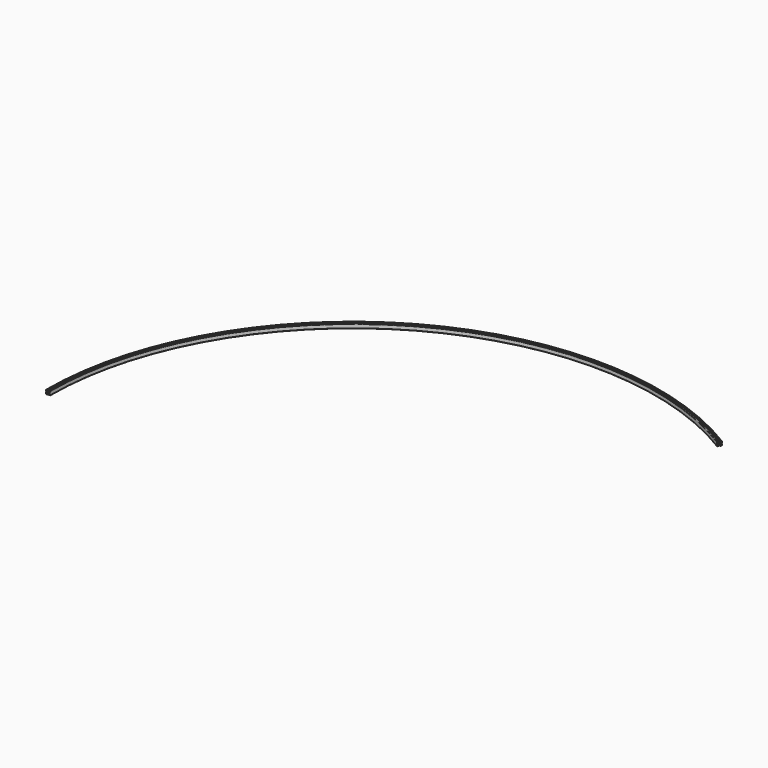
from build123d import *


# Not quite as in the source:
# - ends of sketch curves that miss each other by under 0.0002 mm in the source are joined


with BuildPart() as f2:
    # F2: sweep along a path in F1
    with BuildLine(Plane.XY) as f2_path:
        ThreePointArc((0, 0), (1542.5596027822, 2633.9267022203), (4594.4171342179, 2577.132260378))
    # F0 (on Front) → F2 (sweep)
    with BuildSketch(Plane.XZ):
        with BuildLine():
            Line((20, -17.173511), (20, 17))
            ThreePointArc((20, 17), (19.1213203436, 19.1213203436), (17, 20))
            Line((17, 20), (4.1, 20))
            Line((4.1, 20), (4.1, 17))
            Line((4.1, 17), (10.5, 17))
            Line((10.5, 17), (10.5, 12.662742))
            ThreePointArc((10.5, 12.662742), (10.378207252, 12.0504485082), (10.0313708499, 11.5313711501))
            Line((10.0313708499, 11.5313711501), (8.171573, 9.671573))
            ThreePointArc((8.171573, 9.671573), (6.8738797295, 8.80448187), (5.343146, 8.5))
            Line((5.343146, 8.5), (-5.343146, 8.5))
            ThreePointArc((-5.343146, 8.5), (-6.8738797295, 8.80448187), (-8.1715731247, 9.6715728753))
            Line((-8.1715731247, 9.6715728753), (-10.031371, 11.531371))
            ThreePointArc((-10.031371, 11.531371), (-10.378207252, 12.0504485082), (-10.5, 12.662742))
            Line((-10.5, 12.662742), (-10.5, 17))
            Line((-10.5, 17), (-4.1, 17))
            Line((-4.1, 17), (-4.1, 20))
            Line((-4.1, 20), (-17, 20))
            ThreePointArc((-17, 20), (-19.1213203436, 19.1213203436), (-20, 17))
            Line((-20, 17), (-20, 4.1))
            Line((-20, 4.1), (-17, 4.1))
            Line((-17, 4.1), (-17, 10.5))
            Line((-17, 10.5), (-12.662742, 10.5))
            ThreePointArc((-12.662742, 10.5), (-12.0504485082, 10.378207252), (-11.5313711501, 10.0313708499))
            Line((-11.5313711501, 10.0313708499), (-9.671573, 8.171573))
            ThreePointArc((-9.671573, 8.171573), (-8.80448187, 6.8738797295), (-8.5, 5.343146))
            Line((-8.5, 5.343146), (-8.5, -5.343146))
            ThreePointArc((-8.5, -5.343146), (-8.80448187, -6.8738797295), (-9.6715728753, -8.1715731247))
            Line((-9.6715728753, -8.1715731247), (-11.531371, -10.031371))
            ThreePointArc((-11.531371, -10.031371), (-12.0504485082, -10.378207252), (-12.662742, -10.5))
            Line((-12.662742, -10.5), (-17, -10.5))
            Line((-17, -10.5), (-17, -4.1))
            Line((-17, -4.1), (-20, -4.1))
            Line((-20, -4.1), (-20, -17))
            ThreePointArc((-20, -17), (-19.1213203436, -19.1213203436), (-17, -20))
            Line((-17, -20), (-4.1, -20))
            Line((-4.1, -20), (-4.1, -17))
            Line((-4.1, -17), (-10.5, -17))
            Line((-10.5, -17), (-10.5, -12.662742))
            ThreePointArc((-10.5, -12.662742), (-10.378207252, -12.0504485082), (-10.0313708499, -11.5313711501))
            Line((-10.0313708499, -11.5313711501), (-8.171573, -9.671573))
            ThreePointArc((-8.171573, -9.671573), (-6.8738797295, -8.80448187), (-5.343146, -8.5))
            Line((-5.343146, -8.5), (5.343146, -8.5))
            ThreePointArc((5.343146, -8.5), (6.8738797295, -8.80448187), (8.1715731247, -9.6715728753))
            Line((8.1715731247, -9.6715728753), (10.031371, -11.531371))
            ThreePointArc((10.031371, -11.531371), (10.378207252, -12.0504485082), (10.5, -12.662742))
            Line((10.5, -12.662742), (10.5, -17))
            Line((10.5, -17), (4.1, -17))
            Line((4.1, -17), (4.1, -20))
            Line((4.1, -20), (10.794536, -20))
            ThreePointArc((10.794536, -20), (11.8571230554, -19.5587297813), (12.294526081, -18.4945449997))
            Line((12.294526081, -18.4945449997), (12.281818, -15))
            Line((12.281818, -15), (11.981816, -15))
            Line((11.981816, -15), (11.967271, -11))
            Line((11.967271, -11), (12.267273, -11))
            Line((12.267273, -11), (12.2, 7.5))
            Line((12.2, 7.5), (16.6, 7.5))
            Line((16.6, 7.5), (16.532727, -11))
            Line((16.532727, -11), (16.832729, -11))
            Line((16.832729, -11), (16.818184, -15))
            Line((16.818184, -15), (16.518182, -15))
            Line((16.518182, -15), (16.505474, -18.494545))
            ThreePointArc((16.505474, -18.494545), (16.9428769446, -19.5587297813), (18.005464, -20))
            ThreePointArc((18.005464, -20), (19.4511622088, -18.9031941577), (20, -17.173511))
        make_face()
        with BuildLine():
            ThreePointArc((-17, -18.5), (-18.0606601718, -18.0606601718), (-18.5, -17))
            Line((-18.5, -17), (-18.5, -12))
            Line((-18.5, -12), (-12, -12))
            Line((-12, -12), (-12, -18.5))
            Line((-12, -18.5), (-17, -18.5))
        make_face(mode=Mode.SUBTRACT)
        with BuildLine():
            ThreePointArc((-3.3004280183, 5.0107060277), (-2.268365446, 5.5546843478), (-1.1505419264, 5.8886546236))
            Line((-1.1505419264, 5.8886546236), (-1.150542, 7.15))
            Line((-1.150542, 7.15), (1.150542, 7.15))
            Line((1.150542, 7.15), (1.150542, 5.888655))
            ThreePointArc((1.150542, 5.888655), (2.268365446, 5.5546843478), (3.3004280183, 5.0107060277))
            Line((3.3004280183, 5.0107060277), (4.199561, 5.909838))
            Line((4.199561, 5.909838), (4.199561, 7.15))
            Line((4.199561, 7.15), (9.2, 7.15))
            Line((9.2, 7.15), (9.199992, 4.199561))
            Line((9.199992, 4.199561), (5.909838, 4.199561))
            Line((5.909838, 4.199561), (5.010706, 3.300428))
            ThreePointArc((5.010706, 3.300428), (5.5546843478, 2.268365446), (5.8886546236, 1.1505419264))
            Line((5.8886546236, 1.1505419264), (9.199984, 1.150542))
            Line((9.199984, 1.150542), (9.199978, -1.150542))
            Line((9.199978, -1.150542), (5.888655, -1.150542))
            ThreePointArc((5.888655, -1.150542), (5.5546843478, -2.268365446), (5.0107060277, -3.3004280183))
            Line((5.0107060277, -3.3004280183), (5.909838, -4.199561))
            Line((5.909838, -4.199561), (9.19997, -4.199561))
            Line((9.19997, -4.199561), (9.199961, -7.708938))
            ThreePointArc((9.199961, -7.708938), (8.9307701444, -8.1524753318), (8.4130540825, -8.1184288823))
            ThreePointArc((8.4130540825, -8.1184288823), (6.95266378, -7.3978482465), (5.343146, -7.15))
            Line((5.343146, -7.15), (4.199561, -7.15))
            Line((4.199561, -7.15), (4.199561, -5.909838))
            Line((4.199561, -5.909838), (3.300428, -5.010706))
            ThreePointArc((3.300428, -5.010706), (2.268365446, -5.5546843478), (1.1505419264, -5.8886546236))
            Line((1.1505419264, -5.8886546236), (1.150542, -7.15))
            Line((1.150542, -7.15), (-1.150617, -7.15))
            Line((-1.150617, -7.15), (-1.150617, -5.88864))
            ThreePointArc((-1.150617, -5.88864), (-2.2684008499, -5.5546698898), (-3.3004280183, -5.0107060277))
            Line((-3.3004280183, -5.0107060277), (-4.199561, -5.909838))
            Line((-4.199561, -5.909838), (-4.199561, -7.15))
            Line((-4.199561, -7.15), (-7.15, -7.15))
            Line((-7.15, -7.15), (-7.15, -4.199561))
            Line((-7.15, -4.199561), (-5.909838, -4.199561))
            Line((-5.909838, -4.199561), (-5.010706, -3.300428))
            ThreePointArc((-5.010706, -3.300428), (-5.5546843478, -2.268365446), (-5.8886546236, -1.1505419264))
            Line((-5.8886546236, -1.1505419264), (-7.15, -1.150542))
            Line((-7.15, -1.150542), (-7.15, 1.150542))
            Line((-7.15, 1.150542), (-5.888655, 1.150542))
            ThreePointArc((-5.888655, 1.150542), (-5.5546843478, 2.268365446), (-5.0107060277, 3.3004280183))
            Line((-5.0107060277, 3.3004280183), (-5.909838, 4.199561))
            Line((-5.909838, 4.199561), (-7.15, 4.199561))
            Line((-7.15, 4.199561), (-7.15, 7.15))
            Line((-7.15, 7.15), (-4.199561, 7.15))
            Line((-4.199561, 7.15), (-4.199561, 5.909838))
            Line((-4.199561, 5.909838), (-3.3004280183, 5.0107060277))
        make_face(mode=Mode.SUBTRACT)
        with BuildLine():
            ThreePointArc((-18.5, 17), (-18.0606601718, 18.0606601718), (-17, 18.5))
            Line((-17, 18.5), (-12, 18.5))
            Line((-12, 18.5), (-12, 12))
            Line((-12, 12), (-18.5, 12))
            Line((-18.5, 12), (-18.5, 17))
        make_face(mode=Mode.SUBTRACT)
        with BuildLine():
            ThreePointArc((17, 18.5), (18.0606601718, 18.0606601718), (18.5, 17))
            Line((18.5, 17), (18.5, 12))
            Line((18.5, 12), (12, 12))
            Line((12, 12), (12, 18.5))
            Line((12, 18.5), (17, 18.5))
        make_face(mode=Mode.SUBTRACT)
    sweep(path=f2_path.line)


solid = f2.part
